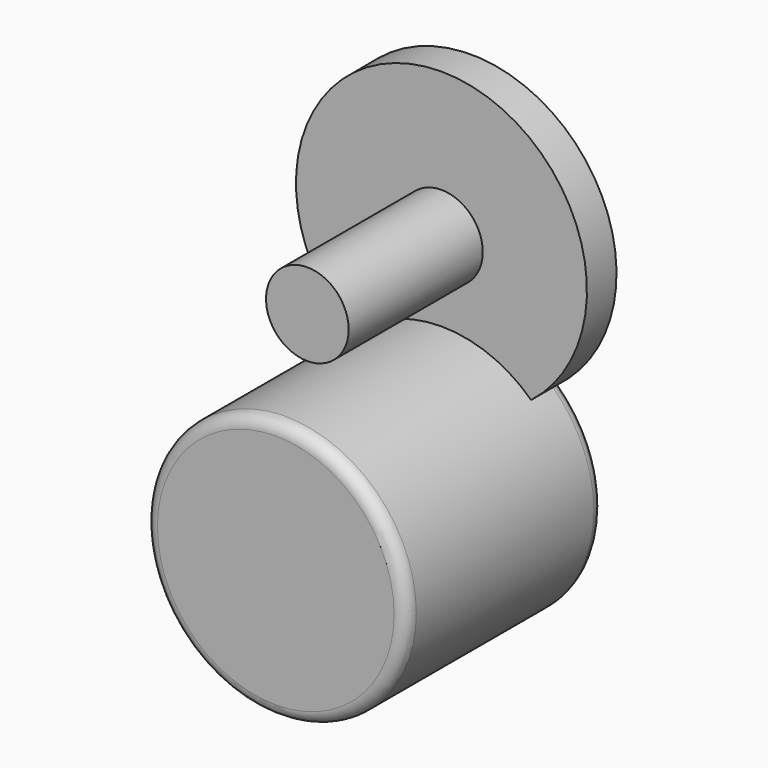
from build123d import *

# Parameters (mm, degrees)
F1_R     = 53
F2_DEPTH = 50
F3_R     = 5
F4_R     = 16.75
F5_DEPTH = 34
F6_R     = 59
F7_DEPTH = 15


with BuildPart() as f2:
    # F1 (on Front) → F2 (new body, symmetric)
    with BuildSketch(Plane.XZ):
        with Locations((0, -85)):
            Circle(F1_R)
    extrude(amount=F2_DEPTH, both=True)

    # F3
    f3_edges = [f2.edges().sort_by_distance(p)[0] for p in [
        (-53, -50, -85),
        (-53, 50, -85),
    ]]
    fillet(f3_edges, radius=F3_R)

    # F6 (on face) → F7 (join)
    with BuildSketch(Plane(origin=(0, 34, 0), x_dir=(-1, 0, 0), z_dir=(0, 1, 0))):
        Circle(F6_R)
    extrude(amount=F7_DEPTH)


with BuildPart() as f5:
    # F4 (on Front) → F5 (new body, symmetric)
    with BuildSketch(Plane.XZ):
        Circle(F4_R)
    extrude(amount=F5_DEPTH, both=True)


solid = Compound([f2.part, f5.part])
